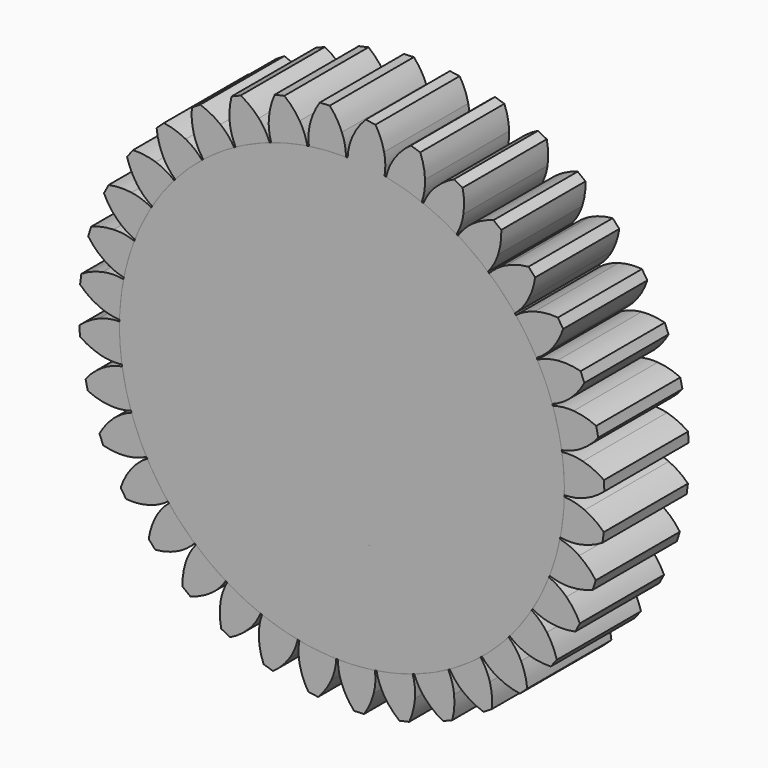
from build123d import *

# Parameters (mm, degrees)
F1_DEPTH = 12.7
F2_COUNT = 36


with BuildPart() as f1:
    # F0 (on Front) → F1 (new body, symmetric)
    with BuildSketch(Plane.XZ):
        with BuildLine():
            ThreePointArc((-7.9757188017, 53.1256411782), (-35.0534039093, -40.7087793402), (53.721, 0))
            ThreePointArc((53.721, 0), (38.329016413, 37.6408334368), (0.9731977694, 53.7121841587))
            ThreePointArc((0.9731977694, 53.7121841587), (-3.5135215054, 53.6059792153), (-7.9757188017, 53.1256411782))
        make_face()
        with BuildLine():
            ThreePointArc((-7.9757188017, 53.1256411782), (-3.5135215054, 53.6059792153), (0.9731977694, 53.7121841587))
            ThreePointArc((0.9731977694, 53.7121841587), (0.7215842218, 56.2391814977), (0, 58.674))
            ThreePointArc((0, 58.674), (-1.2615875471, 61.1535577549), (-2.9383220097, 63.3735513))
            ThreePointArc((-2.9383220097, 63.3735513), (-4.1265686515, 63.3161032649), (-5.315564527, 63.2771267818))
            ThreePointArc((-5.315564527, 63.2771267818), (-6.7155957045, 60.8294795639), (-7.6584938023, 58.1720357962))
            ThreePointArc((-7.6584938023, 58.1720357962), (-8.0560971832, 55.6638618629), (-7.9757188017, 53.1256411782))
        make_face()
    extrude(amount=F1_DEPTH, both=True)


with BuildPart() as f2_1:
    # F2: instance of F1
    add(f1.part.rotate(Axis((0, 0, 0), (0, -1, 0)), 1 * 360 / F2_COUNT))


with BuildPart() as f2_2:
    # F2: instance of F1
    add(f1.part.rotate(Axis((0, 0, 0), (0, -1, 0)), 2 * 360 / F2_COUNT))


with BuildPart() as f2_3:
    # F2: instance of F1
    add(f1.part.rotate(Axis((0, 0, 0), (0, -1, 0)), 3 * 360 / F2_COUNT))


with BuildPart() as f2_4:
    # F2: instance of F1
    add(f1.part.rotate(Axis((0, 0, 0), (0, -1, 0)), 4 * 360 / F2_COUNT))


with BuildPart() as f2_5:
    # F2: instance of F1
    add(f1.part.rotate(Axis((0, 0, 0), (0, -1, 0)), 5 * 360 / F2_COUNT))


with BuildPart() as f2_6:
    # F2: instance of F1
    add(f1.part.rotate(Axis((0, 0, 0), (0, -1, 0)), 6 * 360 / F2_COUNT))


with BuildPart() as f2_7:
    # F2: instance of F1
    add(f1.part.rotate(Axis((0, 0, 0), (0, -1, 0)), 7 * 360 / F2_COUNT))


with BuildPart() as f2_8:
    # F2: instance of F1
    add(f1.part.rotate(Axis((0, 0, 0), (0, -1, 0)), 8 * 360 / F2_COUNT))


with BuildPart() as f2_9:
    # F2: instance of F1
    add(f1.part.rotate(Axis((0, 0, 0), (0, -1, 0)), 9 * 360 / F2_COUNT))


with BuildPart() as f2_10:
    # F2: instance of F1
    add(f1.part.rotate(Axis((0, 0, 0), (0, -1, 0)), 10 * 360 / F2_COUNT))


with BuildPart() as f2_11:
    # F2: instance of F1
    add(f1.part.rotate(Axis((0, 0, 0), (0, -1, 0)), 11 * 360 / F2_COUNT))


with BuildPart() as f2_12:
    # F2: instance of F1
    add(f1.part.rotate(Axis((0, 0, 0), (0, -1, 0)), 12 * 360 / F2_COUNT))


with BuildPart() as f2_13:
    # F2: instance of F1
    add(f1.part.rotate(Axis((0, 0, 0), (0, -1, 0)), 13 * 360 / F2_COUNT))


with BuildPart() as f2_14:
    # F2: instance of F1
    add(f1.part.rotate(Axis((0, 0, 0), (0, -1, 0)), 14 * 360 / F2_COUNT))


with BuildPart() as f2_15:
    # F2: instance of F1
    add(f1.part.rotate(Axis((0, 0, 0), (0, -1, 0)), 15 * 360 / F2_COUNT))


with BuildPart() as f2_16:
    # F2: instance of F1
    add(f1.part.rotate(Axis((0, 0, 0), (0, -1, 0)), 16 * 360 / F2_COUNT))


with BuildPart() as f2_17:
    # F2: instance of F1
    add(f1.part.rotate(Axis((0, 0, 0), (0, -1, 0)), 17 * 360 / F2_COUNT))


with BuildPart() as f2_18:
    # F2: instance of F1
    add(f1.part.rotate(Axis((0, 0, 0), (0, -1, 0)), 18 * 360 / F2_COUNT))


with BuildPart() as f2_19:
    # F2: instance of F1
    add(f1.part.rotate(Axis((0, 0, 0), (0, -1, 0)), 19 * 360 / F2_COUNT))


with BuildPart() as f2_20:
    # F2: instance of F1
    add(f1.part.rotate(Axis((0, 0, 0), (0, -1, 0)), 20 * 360 / F2_COUNT))


with BuildPart() as f2_21:
    # F2: instance of F1
    add(f1.part.rotate(Axis((0, 0, 0), (0, -1, 0)), 21 * 360 / F2_COUNT))


with BuildPart() as f2_22:
    # F2: instance of F1
    add(f1.part.rotate(Axis((0, 0, 0), (0, -1, 0)), 22 * 360 / F2_COUNT))


with BuildPart() as f2_23:
    # F2: instance of F1
    add(f1.part.rotate(Axis((0, 0, 0), (0, -1, 0)), 23 * 360 / F2_COUNT))


with BuildPart() as f2_24:
    # F2: instance of F1
    add(f1.part.rotate(Axis((0, 0, 0), (0, -1, 0)), 24 * 360 / F2_COUNT))


with BuildPart() as f2_25:
    # F2: instance of F1
    add(f1.part.rotate(Axis((0, 0, 0), (0, -1, 0)), 25 * 360 / F2_COUNT))


with BuildPart() as f2_26:
    # F2: instance of F1
    add(f1.part.rotate(Axis((0, 0, 0), (0, -1, 0)), 26 * 360 / F2_COUNT))


with BuildPart() as f2_27:
    # F2: instance of F1
    add(f1.part.rotate(Axis((0, 0, 0), (0, -1, 0)), 27 * 360 / F2_COUNT))


with BuildPart() as f2_28:
    # F2: instance of F1
    add(f1.part.rotate(Axis((0, 0, 0), (0, -1, 0)), 28 * 360 / F2_COUNT))


with BuildPart() as f2_29:
    # F2: instance of F1
    add(f1.part.rotate(Axis((0, 0, 0), (0, -1, 0)), 29 * 360 / F2_COUNT))


with BuildPart() as f2_30:
    # F2: instance of F1
    add(f1.part.rotate(Axis((0, 0, 0), (0, -1, 0)), 30 * 360 / F2_COUNT))


with BuildPart() as f2_31:
    # F2: instance of F1
    add(f1.part.rotate(Axis((0, 0, 0), (0, -1, 0)), 31 * 360 / F2_COUNT))


with BuildPart() as f2_32:
    # F2: instance of F1
    add(f1.part.rotate(Axis((0, 0, 0), (0, -1, 0)), 32 * 360 / F2_COUNT))


with BuildPart() as f2_33:
    # F2: instance of F1
    add(f1.part.rotate(Axis((0, 0, 0), (0, -1, 0)), 33 * 360 / F2_COUNT))


with BuildPart() as f2_34:
    # F2: instance of F1
    add(f1.part.rotate(Axis((0, 0, 0), (0, -1, 0)), 34 * 360 / F2_COUNT))


with BuildPart() as f2_35:
    # F2: instance of F1
    add(f1.part.rotate(Axis((0, 0, 0), (0, -1, 0)), 35 * 360 / F2_COUNT))


solid = Compound([f1.part, f2_1.part, f2_2.part, f2_3.part, f2_4.part, f2_5.part, f2_6.part, f2_7.part, f2_8.part, f2_9.part, f2_10.part, f2_11.part, f2_12.part, f2_13.part, f2_14.part, f2_15.part, f2_16.part, f2_17.part, f2_18.part, f2_19.part, f2_20.part, f2_21.part, f2_22.part, f2_23.part, f2_24.part, f2_25.part, f2_26.part, f2_27.part, f2_28.part, f2_29.part, f2_30.part, f2_31.part, f2_32.part, f2_33.part, f2_34.part, f2_35.part])
